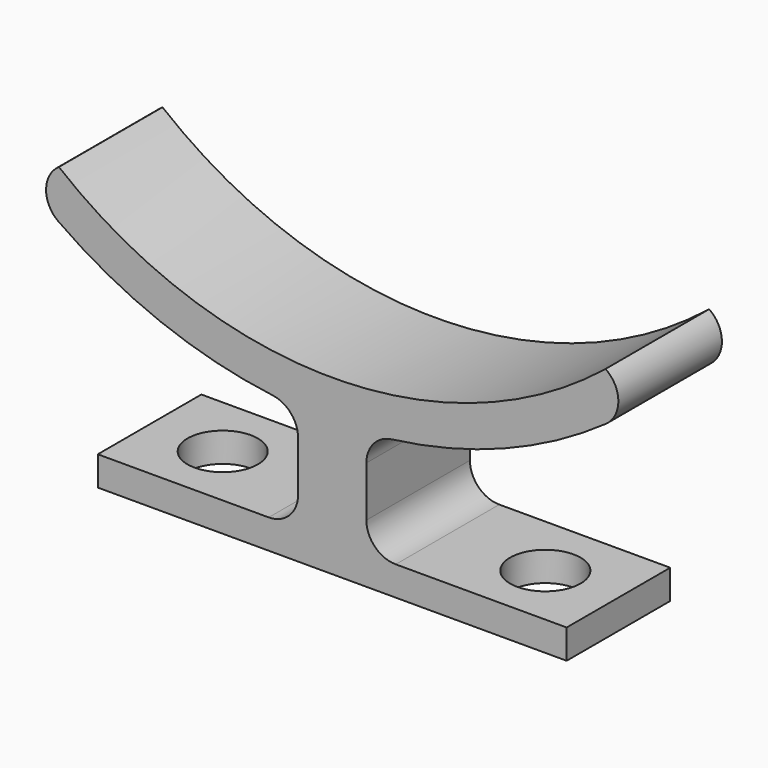
from build123d import *

# Parameters (mm, degrees)
F0_W          = 79.9313783646
F0_H          = 22.0680292696
F0_R          = 6
F1_DEPTH      = 5
F3_DEPTH      = 11.0340146348
F3_DEPTH_BACK = 11.0340146348
F4_T1_DEPTH   = 22.0680292696
F4_T3_DEPTH   = 22.0680292696
F4_T5_DEPTH   = 22.0680292696
F4_T7_DEPTH   = 22.0680292696
F4_T9_DEPTH   = 86.1669063659
F4_T11_DEPTH  = 86.1669063659


# Not quite as in the source:
# - a fillet or chamfer that OpenCascade refuses, or shapes differently, is made with other operations: its cross-section is extruded or revolved along the edge and cut away or added


with BuildPart() as f1:
    # F0 (on Top) → F1 (new body)
    with BuildSketch(Plane.XY):
        Rectangle(F0_W, F0_H)
        with Locations((-27.5, 0)):
            Circle(F0_R, mode=Mode.SUBTRACT)
        with Locations((27.5, 0)):
            Circle(F0_R, mode=Mode.SUBTRACT)
    extrude(amount=F1_DEPTH)

    # F2 (on Front) → F3 (join, two sides)
    with BuildSketch(Plane.XZ) as f3_sk:
        with BuildLine():
            ThreePointArc((-5.8236527257, 29.7265377594), (-27.4373325166, 34.7576861994), (-46.5960713348, 45.9561832249))
            Line((-46.5960713348, 45.9561832249), (-56.5117387286, 45.9561832249))
            ThreePointArc((-56.5117387286, 45.9561832249), (-33.1949461114, 30.0355047329), (-5.8236527257, 23.1106856026))
            Line((-5.8236527257, 23.1106856026), (-5.8236527257, 29.7265377594))
        make_face()
        with BuildLine():
            ThreePointArc((5.8236527257, 29.7265377594), (0, 29.4976123348), (-5.8236527257, 29.7265377594))
            Line((-5.8236527257, 29.7265377594), (-5.8236527257, 23.1106856026))
            ThreePointArc((-5.8236527257, 23.1106856026), (0, 22.900505574), (5.8236527257, 23.1106856026))
            Line((5.8236527257, 23.1106856026), (5.8236527257, 29.7265377594))
        make_face()
        with BuildLine():
            Line((56.5117387285, 45.9561832249), (46.5960713348, 45.9561832249))
            ThreePointArc((46.5960713348, 45.9561832249), (27.4373325166, 34.7576861994), (5.8236527257, 29.7265377594))
            Line((5.8236527257, 29.7265377594), (5.8236527257, 23.1106856026))
            ThreePointArc((5.8236527257, 23.1106856026), (33.1949461114, 30.0355047329), (56.5117387285, 45.9561832249))
        make_face()
        with BuildLine():
            ThreePointArc((5.8236527257, 23.1106856026), (0, 22.900505574), (-5.8236527257, 23.1106856026))
            Line((-5.8236527257, 23.1106856026), (-5.8236527257, 0))
            Line((-5.8236527257, 0), (5.8236527257, 0))
            Line((5.8236527257, 0), (5.8236527257, 23.1106856026))
        make_face()
    extrude(amount=F3_DEPTH)
    extrude(f3_sk.sketch, amount=-F3_DEPTH_BACK)

    # F4: fillet of radius 5 on 6 edges, made by hand

    # F4_s2 → F4_t1 (join)
    with BuildSketch(Plane.XZ.offset(-11.0340146348)):
        with BuildLine():
            ThreePointArc((10.8236527257, 5), (7.2881188197, 6.4644660941), (5.8236527257, 10))
            Line((5.8236527257, 10), (5.8236527257, 5))
            Line((5.8236527257, 5), (10.8236527257, 5))
        make_face()
    extrude(amount=F4_T1_DEPTH)

    # F4_s4 → F4_t3 (join)
    with BuildSketch(Plane.XZ.offset(-11.0340146348)):
        with BuildLine():
            ThreePointArc((10.1927990317, 23.5461016937), (7.0717020017, 21.8910349005), (5.8236527257, 18.5860589906))
            Line((5.8236527257, 18.5860589906), (5.8236527257, 23.1106856026))
            ThreePointArc((5.8236527257, 23.1106856026), (8.0111845889, 23.2987047184), (10.1927990317, 23.5461016937))
        make_face()
    extrude(amount=F4_T3_DEPTH)

    # F4_s6 → F4_t5 (join)
    with BuildSketch(Plane.XZ.offset(-11.0340146348)):
        with BuildLine():
            ThreePointArc((-5.8236527257, 18.5860589906), (-7.0717020017, 21.8910349005), (-10.1927990317, 23.5461016937))
            ThreePointArc((-10.1927990317, 23.5461016937), (-8.0111845889, 23.2987047184), (-5.8236527257, 23.1106856026))
            Line((-5.8236527257, 23.1106856026), (-5.8236527257, 18.5860589906))
        make_face()
    extrude(amount=F4_T5_DEPTH)

    # F4_s8 → F4_t7 (join)
    with BuildSketch(Plane.XZ.offset(-11.0340146348)):
        with BuildLine():
            ThreePointArc((-10.8236527257, 5), (-7.2881188197, 6.4644660941), (-5.8236527257, 10))
            Line((-5.8236527257, 10), (-5.8236527257, 5))
            Line((-5.8236527257, 5), (-10.8236527257, 5))
        make_face()
    extrude(amount=F4_T7_DEPTH)

    # F4_s10 → F4_t9 (cut)
    with BuildSketch(Plane.XZ.offset(-43.083453183)):
        with BuildLine():
            ThreePointArc((46.5960713348, 45.9561832249), (48.7794064532, 41.8686786406), (46.6679769916, 37.743571176))
            ThreePointArc((46.6679769916, 37.743571176), (51.7530210054, 41.6543073723), (56.5117387285, 45.9561832249))
            Line((56.5117387285, 45.9561832249), (46.5960713348, 45.9561832249))
        make_face()
    extrude(amount=F4_T9_DEPTH, mode=Mode.SUBTRACT)

    # F4_s12 → F4_t11 (cut)
    with BuildSketch(Plane.XZ.offset(-43.083453183)):
        with BuildLine():
            ThreePointArc((-46.5960713348, 45.9561832249), (-48.7794064532, 41.8686786406), (-46.6679769916, 37.743571176))
            ThreePointArc((-46.6679769916, 37.743571176), (-51.7530210054, 41.6543073723), (-56.5117387286, 45.9561832249))
            Line((-56.5117387286, 45.9561832249), (-46.5960713348, 45.9561832249))
        make_face()
    extrude(amount=F4_T11_DEPTH, mode=Mode.SUBTRACT)


solid = f1.part
